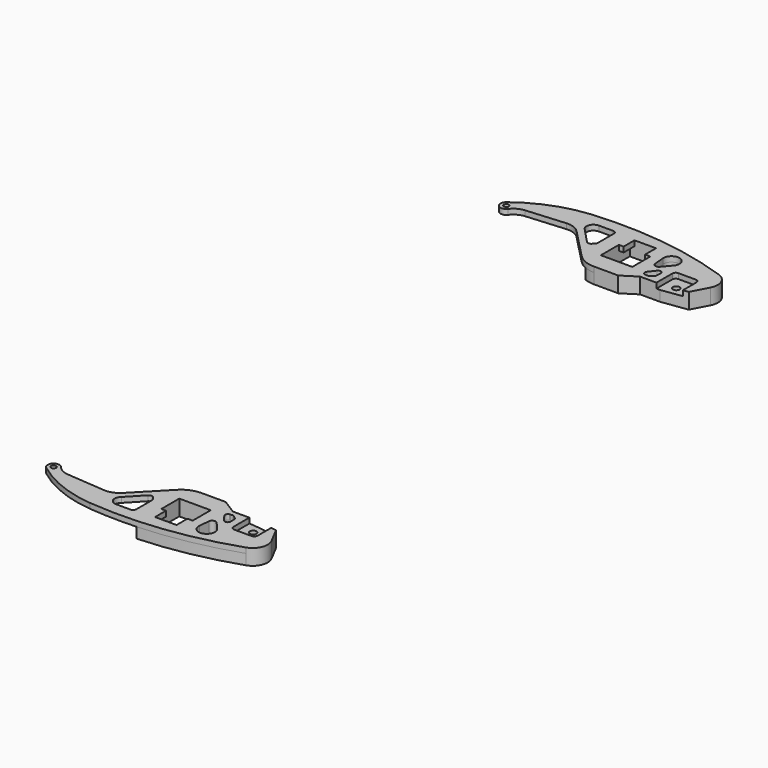
from build123d import *
from build123d import SkipClean  # not in build123d's __all__

# Parameters (mm, degrees)
F0_R     = 1.27
F0_R_2   = 0.9525
F1_DEPTH = 1.9812
F2_W     = 11.9223818183
F2_H     = 13.7107372284
F2_R     = 1.27
F3_DEPTH = 3.9624
F5_DEPTH = 1.9812


# Not quite as in the source:
# - after a boolean that leaves OpenCascade's solid faulty, fix() repairs it


with BuildPart() as f1:
    # F0 (on Top) → F1 (new body)
    with BuildSketch(Plane.XY):
        with BuildLine():
            Line((-47.9935594662, 92.9018468329), (-38.7711464414, 92.9018468329))
            Line((-38.7711464414, 92.9018468329), (-33.2755186414, 96.3824086013))
            Line((-33.2755186414, 96.3824086013), (-25.6948654508, 96.3824086013))
            Line((-25.6948654508, 96.3824086013), (-15.8810783178, 97.7427214384))
            Line((-15.8810783178, 97.7427214384), (-12.636416007, 103.9167105482))
            ThreePointArc((-12.636416007, 103.9167105482), (-12.3860869147, 108.6525727702), (-15.8187403188, 111.9248726108))
            ThreePointArc((-15.8187403188, 111.9248726108), (-42.408191436, 118.0267426348), (-69.6853622794, 118.4599623084))
            ThreePointArc((-69.6853622794, 118.4599623084), (-82.4742788904, 115.4278151789), (-93.9159779713, 108.9595985437))
            ThreePointArc((-93.9159779713, 108.9595985437), (-94.1293035133, 105.6362591622), (-90.8067524433, 105.8615297079))
            ThreePointArc((-90.8067524433, 105.8615297079), (-88.8335264193, 107.5549552633), (-86.3416423602, 108.2978044339))
            Line((-86.3416423602, 108.2978044339), (-71.653987872, 109.474757484))
            ThreePointArc((-71.653987872, 109.474757484), (-68.6729520146, 109.0541017361), (-66.1555117331, 107.4030352715))
            Line((-66.1555117331, 107.4030352715), (-54.9410246313, 95.841743052))
            ThreePointArc((-54.9410246313, 95.841743052), (-51.7655039912, 93.6670703781), (-47.9935594662, 92.9018468329))
        make_face()
        with BuildLine():
            ThreePointArc((-31.729853951, 102.5358076193), (-30.5288188939, 102.8743550973), (-29.8086822236, 101.8552855317))
            ThreePointArc((-29.8086822236, 101.8552855317), (-29.8087704345, 101.8414752371), (-29.8090350527, 101.8276671962))
            Line((-29.8090350527, 101.8276671962), (-29.852613442, 100.1223570045))
            ThreePointArc((-29.852613442, 100.1223570045), (-29.8470387538, 100.0699346624), (-29.8451774306, 100.0172496117))
            ThreePointArc((-29.8451774306, 100.0172496117), (-29.9140658389, 99.7040195755), (-30.1080177856, 99.4485957889))
            Line((-30.1080177856, 99.4485957889), (-31.318617745, 98.418811003))
            ThreePointArc((-31.318617745, 98.418811003), (-31.5535333525, 98.285914355), (-31.821401526, 98.2528461926))
            Line((-31.821401526, 98.2528461926), (-32.6937066692, 98.3167908194))
            ThreePointArc((-32.6937066692, 98.3167908194), (-32.8317059691, 98.3180750151), (-32.9684173403, 98.336928579))
            ThreePointArc((-32.9684173403, 98.336928579), (-33.7642168357, 99.014754834), (-33.6142944517, 100.0492926766))
            Line((-33.6142944517, 100.0492926766), (-31.7720925497, 102.4800738847))
            ThreePointArc((-31.7720925497, 102.4800738847), (-31.751424005, 102.5082823627), (-31.729853951, 102.5358076193))
        make_face(mode=Mode.SUBTRACT)
        with Locations((-22.5797742605, 100.1924086013)):
            Circle(F0_R, mode=Mode.SUBTRACT)
        with Locations((-92.566716894, 107.2044729315)):
            Circle(F0_R_2, mode=Mode.SUBTRACT)
        with BuildLine():
            ThreePointArc((-57.7795208585, 114.3099591136), (-56.8814952464, 113.9379847257), (-56.5095208585, 113.0399591136))
            Line((-56.5095208585, 113.0399591136), (-56.5095208585, 105.5245197072))
            ThreePointArc((-56.5095208585, 105.5245197072), (-56.5940696416, 105.0688823379), (-56.8364585157, 104.6739120317))
            Line((-56.8364585157, 104.6739120317), (-57.5123382575, 103.924569237))
            ThreePointArc((-57.5123382575, 103.924569237), (-58.4388736983, 103.5052844519), (-59.3760069692, 103.9003146871))
            Line((-59.3760069692, 103.9003146871), (-64.8223236203, 109.6314042807))
            ThreePointArc((-64.8223236203, 109.6314042807), (-65.6702235375, 112.5495796966), (-63.193179667, 114.3099591136))
            Line((-63.193179667, 114.3099591136), (-57.7795208585, 114.3099591136))
        make_face(mode=Mode.SUBTRACT)
        Polygon((-40.933508426, 108.3481609821), (-38.946442306, 108.3481609821), (-38.946442306, 99.8037904501), (-50.8688241243, 99.8037904501), (-50.8688241243, 108.3481609821), (-49.0804649889, 108.3481609821), (-49.0804649889, 113.5145276785), (-40.933508426, 113.5145276785), align=None, mode=Mode.SUBTRACT)
        with BuildLine():
            ThreePointArc((-35.3233501937, 109.7291281762), (-32.4270965422, 113.0506303681), (-29.2408396166, 110.0062209297))
            ThreePointArc((-29.2408396166, 110.0062209297), (-29.3876130121, 109.0718435745), (-29.8137957369, 108.2274670254))
            ThreePointArc((-29.8137957369, 108.2274670254), (-29.9624421423, 108.0370704325), (-30.1257006344, 107.8590443638))
            Line((-30.1257006344, 107.8590443638), (-32.5888625406, 104.9495528088))
            ThreePointArc((-32.5888625406, 104.9495528088), (-34.0204329464, 104.5359221908), (-34.9551612301, 105.6964251639))
            Line((-34.9551612301, 105.6964251639), (-35.3233501937, 109.7291281762))
        make_face(mode=Mode.SUBTRACT)
    extrude(amount=F1_DEPTH)

    # F2 (on face) → F3 (join)
    with BuildSketch(Plane(origin=(0, 0, 0), x_dir=(1, 0, 0), z_dir=(0, 0, -1))):
        with BuildLine():
            ThreePointArc((-15.8187403188, -111.9248726108), (-12.3860869147, -108.6525727702), (-12.636416007, -103.9167105482))
            Line((-12.636416007, -103.9167105482), (-15.8810783178, -97.7427214384))
            Line((-15.8810783178, -97.7427214384), (-25.6948654508, -96.3824086013))
            Line((-25.6948654508, -96.3824086013), (-33.2755186414, -96.3824086013))
            Line((-33.2755186414, -96.3824086013), (-38.7711464414, -92.9018468329))
            Line((-38.7711464414, -92.9018468329), (-47.9935594662, -92.9018468329))
            ThreePointArc((-47.9935594662, -92.9018468329), (-49.9815784423, -93.1082123487), (-51.8848241243, -93.7185090381))
            Line((-51.8848241243, -93.7185090381), (-51.8848241243, -118.8269193207))
            ThreePointArc((-51.8848241243, -118.8269193207), (-33.6074883899, -116.652433517), (-15.8187403188, -111.9248726108))
        make_face()
        with Locations((-44.9076332152, -106.6591590643)):
            Rectangle(F2_W, F2_H, mode=Mode.SUBTRACT)
        with BuildLine():
            Line((-32.5888625406, -104.9495528088), (-30.1257006344, -107.8590443638))
            ThreePointArc((-30.1257006344, -107.8590443638), (-31.2566588837, -112.873826319), (-35.3233501937, -109.7291281762))
            Line((-35.3233501937, -109.7291281762), (-34.9551612301, -105.6964251639))
            ThreePointArc((-34.9551612301, -105.6964251639), (-34.0204329464, -104.5359221908), (-32.5888625406, -104.9495528088))
        make_face(mode=Mode.SUBTRACT)
        with BuildLine():
            ThreePointArc((-29.8090350527, -101.8276671962), (-30.5488332951, -102.8812249507), (-31.7720925497, -102.4800738847))
            Line((-31.7720925497, -102.4800738847), (-33.6142944517, -100.0492926766))
            ThreePointArc((-33.6142944517, -100.0492926766), (-33.7073705562, -98.8890012798), (-32.6937066692, -98.3167908194))
            Line((-32.6937066692, -98.3167908194), (-31.821401526, -98.2528461926))
            ThreePointArc((-31.821401526, -98.2528461926), (-31.5535333525, -98.285914355), (-31.318617745, -98.418811003))
            Line((-31.318617745, -98.418811003), (-30.1080177856, -99.4485957889))
            ThreePointArc((-30.1080177856, -99.4485957889), (-29.8936506369, -99.7526240879), (-29.852613442, -100.1223570045))
            Line((-29.852613442, -100.1223570045), (-29.8090350527, -101.8276671962))
        make_face(mode=Mode.SUBTRACT)
        with Locations((-22.5797742605, -100.1924086013)):
            Circle(F2_R, mode=Mode.SUBTRACT)
    with SkipClean():  # cleaning this boolean's faces spoils the solid; the shape is the same uncleaned
        extrude(amount=F3_DEPTH)

    # F4 (on face) → F5 (cut)
    with BuildSketch(Plane.XY.offset(1.9812)):
        with BuildLine():
            Line((-27.0608905703, 103.9116269755), (-27.0608905703, 96.3824086013))
            Line((-27.0608905703, 96.3824086013), (-25.6948654508, 96.3824086013))
            Line((-25.6948654508, 96.3824086013), (-17.9199781269, 97.4601045907))
            Line((-17.9199781269, 97.4601045907), (-17.9199781269, 103.9116269755))
            ThreePointArc((-17.9199781269, 103.9116269755), (-18.2919525148, 104.8096525876), (-19.1899781269, 105.1816269755))
            Line((-19.1899781269, 105.1816269755), (-25.7908905703, 105.1816269755))
            ThreePointArc((-25.7908905703, 105.1816269755), (-26.6889161824, 104.8096525876), (-27.0608905703, 103.9116269755))
        make_face()
    extrude(amount=-F5_DEPTH, mode=Mode.SUBTRACT)

    add(f1.part.fix(), mode=Mode.REPLACE)


with BuildPart() as f6_1:
    # F6: instance of F1
    add(f1.part.mirror(Plane.XZ), clean=False)


solid = Compound([f1.part, f6_1.part])
